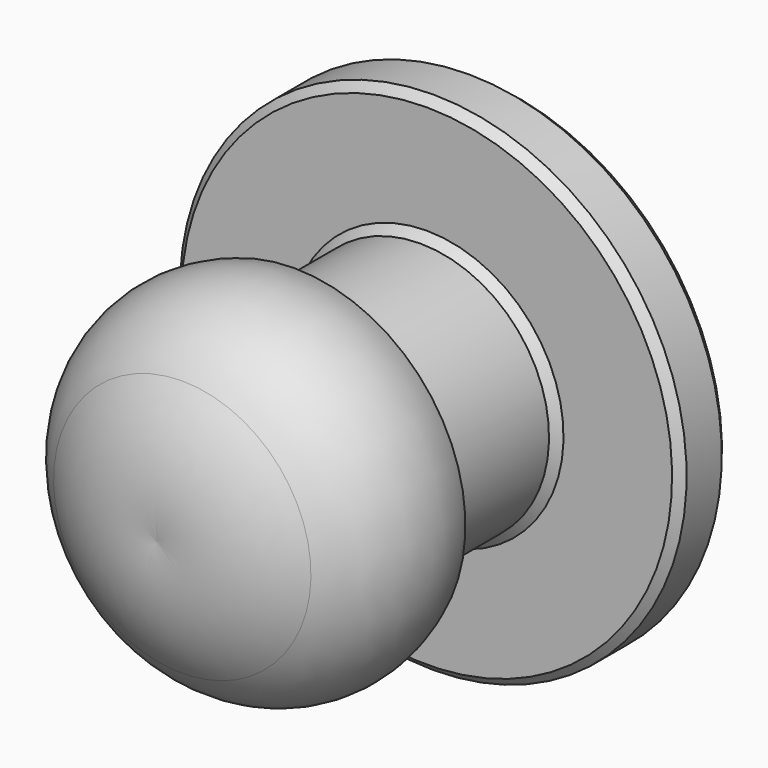
from build123d import *


# Not quite as in the source:
# - a fillet or chamfer that OpenCascade refuses, or shapes differently, is made with other operations: its cross-section is extruded or revolved along the edge and cut away or added


with BuildPart() as f1:
    # F0 (on Right) → F1 (revolve)
    with BuildSketch(Plane.YZ):
        with BuildLine():
            Line((-1, 1.05), (0, 1.05))
            Line((0, 1.05), (3, 1.05))
            ThreePointArc((3, 1.05), (2.9307123176, 2.1090277533), (2.7240305654, 3.15))
            Line((2.7240305654, 3.15), (2, 3.15))
            Line((2, 3.15), (2, 1.6))
            Line((2, 1.6), (0, 1.6))
            Line((0, 1.6), (0, 2.1))
            ThreePointArc((0, 2.1), (-0.9955936413, 2.1941371089), (-1.8, 1.6))
            ThreePointArc((-1.8, 1.6), (-2.1556032846, 0.8389008212), (-2.2, 0))
            Line((-2.2, 0), (-1, 0))
            Line((-1, 0), (-1, 1.05))
        make_face()
    revolve(axis=Axis((0, -1.6, 0), (0, -1, 0)))

    # F2: chamfer of 0.1 on 5 edges, made by hand

    # F2_s1 → F2_t2 (revolve)
    with BuildSketch(Plane.YZ):
        Polygon((2, 1.7), (1.9, 1.6), (2, 1.6), align=None)
    revolve(axis=Axis((0, 2, 0), (0, -1, 0)))

    # F2_s3 → F2_t4 (revolve)
    with BuildSketch(Plane.YZ):
        Polygon((0.1, 1.6), (0, 1.7), (0, 1.6), align=None)
    revolve(axis=Axis((0, 0, 0), (0, -1, 0)))

    # F2_s5 → F2_t6 (revolve, cut)
    with BuildSketch(Plane.YZ):
        Polygon((2.1, 3.15), (2, 3.05), (2, 3.15), align=None)
    revolve(axis=Axis((0, 2, 0), (0, -1, 0)), mode=Mode.SUBTRACT)

    # F2_s7 → F2_t8 (revolve, cut)
    with BuildSketch(Plane.YZ):
        with BuildLine():
            Line((0, 2.0362919162), (-0.0599313668, 2.1279134455))
            ThreePointArc((-0.0599313668, 2.1279134455), (-0.0313408369, 2.1150266488), (0, 2.1))
            Line((0, 2.1), (0, 2.0362919162))
        make_face()
    revolve(axis=Axis((0, 0, 0), (0, -1, 0)), mode=Mode.SUBTRACT)

    # F2_s9 → F2_t10 (revolve, cut)
    with BuildSketch(Plane.YZ):
        with BuildLine():
            Line((2.7437286622, 3.0749128052), (2.6468816068, 3.15))
            Line((2.6468816068, 3.15), (2.7240305654, 3.15))
            ThreePointArc((2.7240305654, 3.15), (2.734371605, 3.1109455948), (2.7437286622, 3.0749128052))
        make_face()
    revolve(axis=Axis((0, 2.7240305654, 0), (0, -1, 0)), mode=Mode.SUBTRACT)


solid = f1.part
